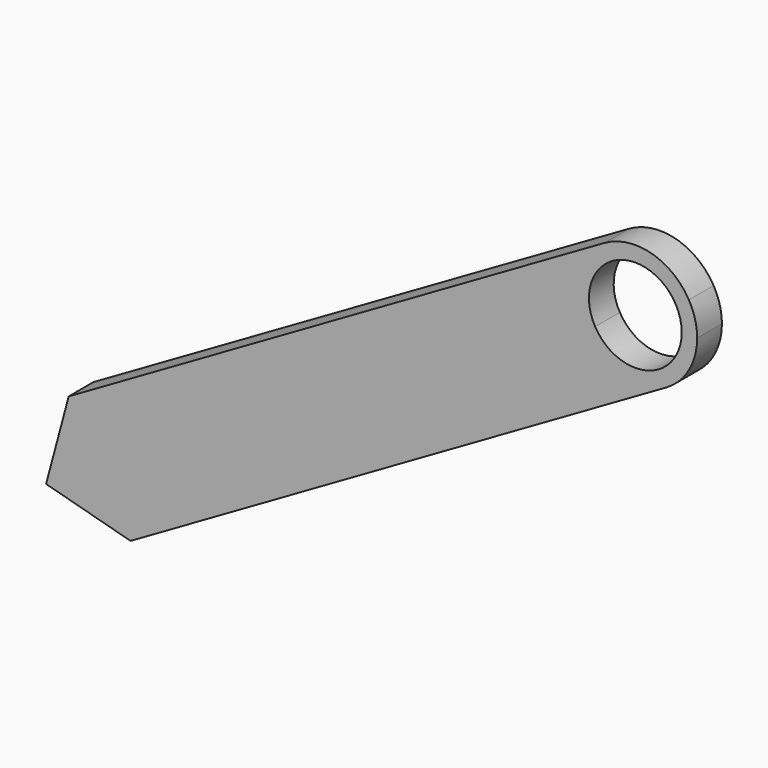
from build123d import *

# Parameters (mm, degrees)
F1_DEPTH = 3.175


with BuildPart() as f1:
    # F0 (on Front) → F1 (new body, symmetric)
    with BuildSketch(Plane.XZ):
        with BuildLine():
            Line((-109.985226, -63.5), (-10.998523, -6.35))
            ThreePointArc((-10.998523, -6.35), (-12.267258, 3.287002), (-6.35, 10.998523))
            Line((-6.35, 10.998523), (-116.335226, -52.501477))
            Line((-116.335226, -52.501477), (-109.985226, -63.5))
        make_face()
        with BuildLine():
            ThreePointArc((-6.35, 10.998523), (-12.267258, 3.287002), (-10.998523, -6.35))
            Line((-10.998523, -6.35), (-8.248892, -4.7625))
            ThreePointArc((-8.248892, -4.7625), (-2.465251, 9.200443), (9.525, 0))
            ThreePointArc((9.525, 0), (8.248892, -4.7625), (4.7625, -8.248892))
            Line((4.7625, -8.248892), (6.35, -10.998523))
            ThreePointArc((6.35, -10.998523), (10.998523, -6.35), (12.7, 0))
            ThreePointArc((12.7, 0), (12.267258, 3.287002), (10.998523, 6.35))
            ThreePointArc((10.998523, 6.35), (3.287002, 12.267258), (-6.35, 10.998523))
        make_face()
        with BuildLine():
            Line((-8.248892, -4.7625), (-10.998523, -6.35))
            ThreePointArc((-10.998523, -6.35), (-3.287002, -12.267258), (6.35, -10.998523))
            Line((6.35, -10.998523), (4.7625, -8.248892))
            ThreePointArc((4.7625, -8.248892), (-2.465251, -9.200443), (-8.248892, -4.7625))
        make_face()
        with BuildLine():
            Line((-10.998523, -6.35), (-4.648523, -17.348523))
            Line((-4.648523, -17.348523), (6.35, -10.998523))
            ThreePointArc((6.35, -10.998523), (-3.287002, -12.267258), (-10.998523, -6.35))
        make_face()
        Polygon((-103.635226, -74.498523), (-4.648523, -17.348523), (-10.998523, -6.35), (-109.985226, -63.5), align=None)
        Polygon((-120.983749, -69.85), (-109.985226, -63.5), (-116.335226, -52.501477), align=None)
        Polygon((-120.983749, -69.85), (-103.635226, -74.498523), (-109.985226, -63.5), align=None)
    extrude(amount=F1_DEPTH, both=True)


solid = f1.part
